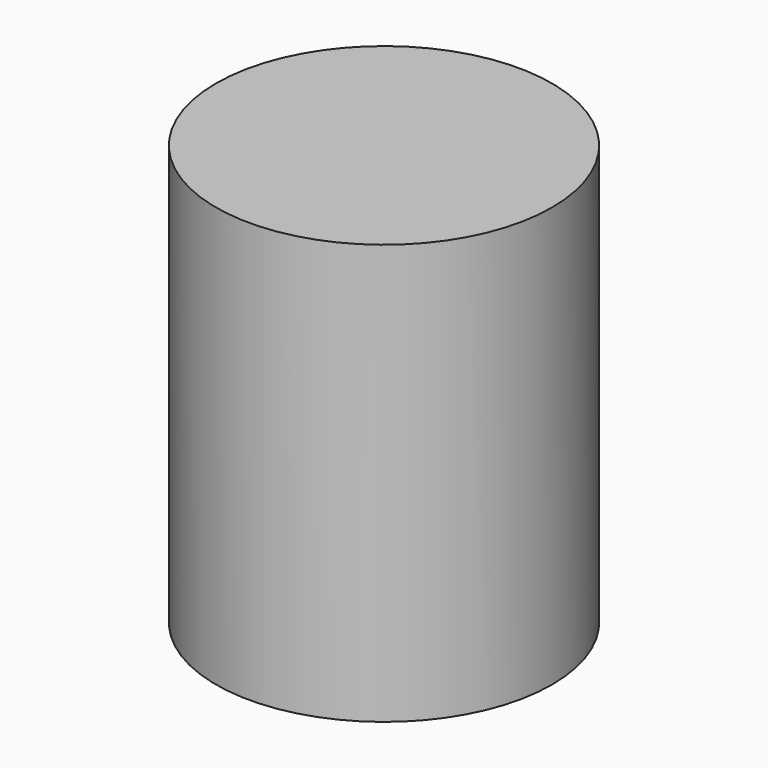
from build123d import *

# Parameters (mm, degrees)
F0_R     = 4.7625
F1_DEPTH = 11.90625


# Not quite as in the source:
# - a length typed as a fraction of an inch, garbled in the dataset ("3 / 203.2 mm" for 3/8 in), is restored


with BuildPart() as f1:
    # F0 (on Top) → F1 (new body)
    with BuildSketch(Plane.XY):
        Circle(F0_R)
    extrude(amount=F1_DEPTH)


solid = f1.part
